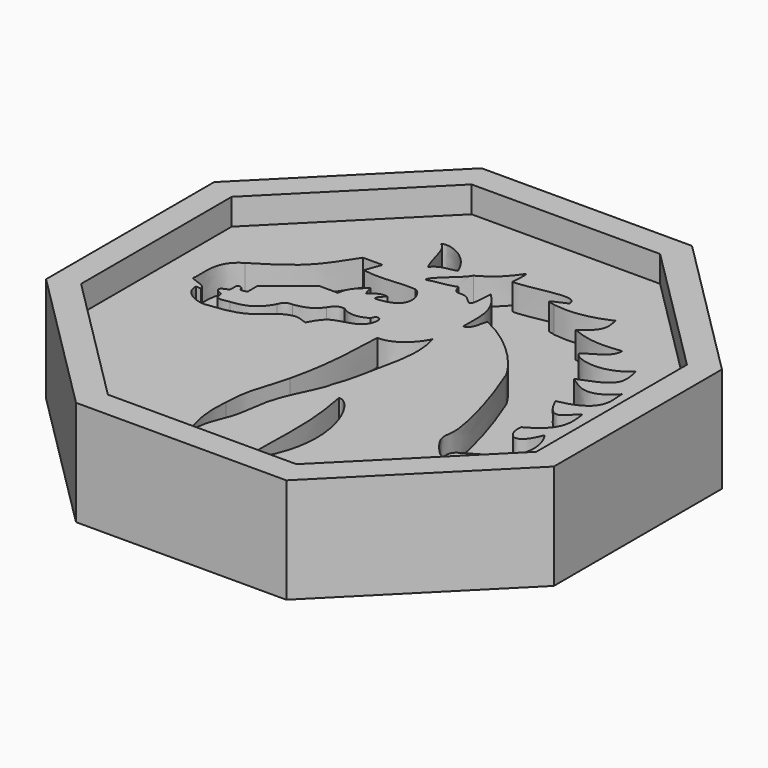
from build123d import *

# Parameters (mm, degrees)
F1_DEPTH = 25.4
F3_DEPTH = 6.35
F5_DEPTH = 6.35


with BuildPart() as f1:
    # F0 (on Top) → F1 (new body)
    with BuildSketch(Plane.XY):
        Polygon((-61.3372846899, 25.3607087968), (-61.3047391097, -25.4392807779), (-25.3607087968, -61.3372846899), (25.4392807779, -61.3047391097), (61.3372846899, -25.3607087968), (61.3047391097, 25.4392807779), (25.3607087968, 61.3372846899), (-25.4392807779, 61.3047391097), align=None)
    extrude(amount=F1_DEPTH)

    # F2 (on face) → F3 (cut)
    with BuildSketch(Plane.XY.offset(25.4)):
        Polygon((-54.9856008905, 22.734521413), (-54.9564255154, -22.8049569991), (-22.734521413, -54.9856008905), (22.8049569991, -54.9564255154), (54.9856008905, -22.734521413), (54.9564255154, 22.8049569991), (22.734521413, 54.9856008905), (-22.8049569991, 54.9564255154), align=None)
    extrude(amount=-F3_DEPTH, mode=Mode.SUBTRACT)

    # F4 (on face) → F5 (cut)
    with BuildSketch(Plane.XY.offset(19.05)):
        with BuildLine():
            add(Edge.make_bspline(
                [(-5.153701175, 4.4508399442), (-0.833334052, 4.1849701665), (2.5564921089, 8.5718045011), (3.3540986478, 10.5658201501)],
                knots=[0, 0, 0, 0, 10.4773871143, 10.4773871143, 10.4773871143, 10.4773871143], degree=3))
            add(Edge.make_bspline(
                [(-5.153701175, 4.4508399442), (-5.4195700213, -3.591689514), (-5.6189713068, -9.9060712382), (-7.679454051, -18.7462065369)],
                knots=[0, 0, 0, 0, 23.3341465033, 23.3341465033, 23.3341465033, 23.3341465033], degree=3))
            add(Edge.make_bspline(
                [(-7.679454051, -18.7462065369), (-9.0719601139, -24.574264884), (-10.8464211226, -26.8810596317), (-11.023866944, -33.9789055288)],
                knots=[0, 0, 0, 0, 15.5955191057, 15.5955191057, 15.5955191057, 15.5955191057], degree=3))
            add(Edge.make_bspline(
                [(-11.023866944, -33.9789055288), (-11.5562053397, -39.74590078), (-10.4887805988, -43.8993513545), (-9.1579346096, -47.1821032425)],
                knots=[0, 0, 0, 0, 13.3343966247, 13.3343966247, 13.3343966247, 13.3343966247], degree=3))
            add(Edge.make_bspline(
                [(-9.1579346096, -47.1821032425), (-8.9959710334, -45.6156823817), (-8.6717623007, -42.2462205811), (-5.5329473264, -35.9645421954), (-5.7178687316, -27.1594780558), (0, -17.6881060287), (0, -15.9681290388)],
                knots=[0, 0, 0, 0, 0.1950520786, 0.422268383, 0.6975815763, 1, 1, 1, 1], degree=3))
            add(Edge.make_bspline(
                [(0, -15.9681290388), (1.8409744371, -11.531976983), (2.5640691165, -5.3227096796), (3.7928808015, 0)],
                knots=[0, 0, 0, 0, 16.4124065808, 16.4124065808, 16.4124065808, 16.4124065808], degree=3))
            add(Edge.make_bspline(
                [(3.3540986478, 10.5658201501), (4.7499099746, 5.580781959), (4.0587496478, 3.0550297815), (3.7928808015, 0)],
                knots=[0, 0, 0, 0, 10.574927197, 10.574927197, 10.574927197, 10.574927197], degree=3))
        make_face()
        with BuildLine():
            add(Edge.make_bspline(
                [(-43.7936633825, 12.6927187666), (-33.5904657841, 18.7789648771), (-32.7022336423, 20.7330770791), (-27.7281291783, 28.312664479)],
                knots=[0, 0, 0, 0, 22.4072330582, 22.4072330582, 22.4072330582, 22.4072330582], degree=3))
            add(Edge.make_bspline(
                [(-43.7936633825, 12.6927187666), (-49.2439717054, 9.5687611029), (-46.8511544168, 3.2543782145), (-47.6487614214, 1.7921003746)],
                knots=[0, 0, 0, 0, 11.5622343091, 11.5622343091, 11.5622343091, 11.5622343091], degree=3))
            add(Edge.make_bspline(
                [(-47.6487614214, 1.7921003746), (-46.3637287418, 0.9944941849), (-43.7936633825, 0.7950926083), (-43.7936633825, -0.6007181946)],
                knots=[0, 0, 0, 0, 4.5373297869, 4.5373297869, 4.5373297869, 4.5373297869], degree=3))
            add(Edge.make_bspline(
                [(-43.7936633825, -0.6007181946), (-44.1924668849, -0.6007181946), (-44.5912703872, -0.6007181946), (-44.9900738895, -0.6007181946)],
                knots=[0, 0, 0, 0, 1.196410507, 1.196410507, 1.196410507, 1.196410507], degree=3))
            add(Edge.make_bspline(
                [(-44.9900738895, -0.6007181946), (-45.1230071485, -4.1899462231), (-40.1379652321, -5.6522237137), (-38.5427549481, -5.1204864867)],
                knots=[0, 0, 0, 0, 7.8737682812, 7.8737682812, 7.8737682812, 7.8737682812], degree=3))
            add(Edge.make_bspline(
                [(-38.5427549481, -5.1204864867), (-27.9080048203, -4.2564133182), (-29.1930399835, -0.9552098345), (-24.451714009, 1.1274284916)],
                knots=[0, 0, 0, 0, 15.4140804566, 15.4140804566, 15.4140804566, 15.4140804566], degree=3))
            add(Edge.make_bspline(
                [(-24.451714009, 1.1274284916), (-21.6600932181, 2.25737039), (-21.2264427294, 1.0571385501), (-19.6755416691, 0.8798926719)],
                knots=[0, 0, 0, 0, 4.7825825871, 4.7825825871, 4.7825825871, 4.7825825871], degree=3))
            add(Edge.make_bspline(
                [(-19.6755416691, 0.8798926719), (-17.4190271646, 5.053767818), (-16.5865225717, 4.7882171348), (-13.464611955, 5.7733519934)],
                knots=[0, 0, 0, 0, 7.9070596333, 7.9070596333, 7.9070596333, 7.9070596333], degree=3))
            add(Edge.make_bspline(
                [(-13.464611955, 5.7733519934), (-9.7631495446, 6.7144022323), (-9.5122028142, 9.0983957052), (-9.4494661316, 9.9139725789)],
                knots=[0, 0, 0, 0, 5.7676801936, 5.7676801936, 5.7676801936, 5.7676801936], degree=3))
            add(Edge.make_bspline(
                [(-9.4494661316, 9.9139725789), (-9.5130050048, 10.6128992403), (-10.0662827589, 11.2702429195), (-11.0193404401, 10.7820779901), (-11.1433556303, 9.9139725789)],
                knots=[0, 0, 0, 0, 0.4822181439, 1, 1, 1, 1], degree=3))
            add(Edge.make_bspline(
                [(-11.1433556303, 9.9139725789), (-12.0216691867, 9.4748158008), (-14.7193456069, 7.9063987359), (-17.4170229584, 9.9139725789)],
                knots=[0, 0, 0, 0, 6.2736673281, 6.2736673281, 6.2736673281, 6.2736673281], degree=3))
            add(Edge.make_bspline(
                [(-17.4170229584, 9.9139725789), (-18.2325989008, 9.9139725789), (-19.1109124571, 10.2903926745), (-20.4283818603, 8.1573463976)],
                knots=[0, 0, 0, 0, 3.4862613179, 3.4862613179, 3.4862613179, 3.4862613179], degree=3))
            add(Edge.make_bspline(
                [(-20.4283818603, 8.1573463976), (-21.745853126, 6.2752454542), (-23.3142692596, 5.5224061944), (-26.137419045, 5.0832494162)],
                knots=[0, 0, 0, 0, 6.4840710844, 6.4840710844, 6.4840710844, 6.4840710844], degree=3))
            add(Edge.make_bspline(
                [(-26.137419045, 5.0832494162), (-27.1412041038, 5.1459865645), (-28.144992888, 4.6440928709), (-28.5214129835, 3.3893594518)],
                knots=[0, 0, 0, 0, 2.9244983007, 2.9244983007, 2.9244983007, 2.9244983007], degree=3))
            add(Edge.make_bspline(
                [(-28.5214129835, 3.3893594518), (-30.5917225778, -0.5003142287), (-33.2266651094, -1.12768088), (-36.0498130322, -1.441364293)],
                knots=[0, 0, 0, 0, 8.9449817882, 8.9449817882, 8.9449817882, 8.9449817882], degree=3))
            add(Edge.make_bspline(
                [(-36.0498130322, -1.441364293), (-37.4036222083, -1.7066936684), (-39.5547804741, -2.1193183366), (-39.0422801094, 0.3359437743), (-40.8038466022, 0.3445137653), (-41.1962555545, 1.9460313525), (-38.8704378187, 2.1547470128), (-39.2634177998, 3.7380327234), (-39.1247228012, 4.7924157188), (-37.7836521987, 4.5584381006), (-37.7563586264, 3.2850185978), (-36.639120561, 3.6665562247), (-36.0498130322, 3.8912522141)],
                knots=[0, 0, 0, 0, 0.1488425547, 0.2535303118, 0.353105288, 0.4397851276, 0.5520245867, 0.6506971423, 0.7299289356, 0.813954275, 0.8940290279, 1, 1, 1, 1], degree=3))
            add(Edge.make_bspline(
                [(-36.0498130322, 3.8912522141), (-36.0498130322, 4.7486534653), (-36.0498130322, 5.9197376637), (-36.0498130322, 6.7771389149)],
                knots=[0, 0, 0, 0, 2.8858867008, 2.8858867008, 2.8858867008, 2.8858867008], degree=3))
            add(Edge.make_bspline(
                [(-36.0498130322, 6.7771389149), (-32.9757171373, 9.3284300528), (-30.0270927449, 11.5660382435), (-26.95299685, 14.1173293814)],
                knots=[0, 0, 0, 0, 11.6889033162, 11.6889033162, 11.6889033162, 11.6889033162], degree=3))
            add(Edge.make_bspline(
                [(-26.95299685, 14.1173293814), (-25.3845794747, 14.1173293814), (-23.9938100179, 14.1173293814), (-22.4253926426, 14.1173293814)],
                knots=[0, 0, 0, 0, 4.5276042074, 4.5276042074, 4.5276042074, 4.5276042074], degree=3))
            add(Edge.make_bspline(
                [(-22.4253926426, 14.1173293814), (-22.2210865468, 17.0617159456), (-19.9708938599, 18.3644555509), (-18.9050156623, 19.489550963)],
                knots=[0, 0, 0, 0, 6.4229135761, 6.4229135761, 6.4229135761, 6.4229135761], degree=3))
            add(Edge.make_bspline(
                [(-18.9050156623, 19.489550963), (-18.5299832374, 18.8184417784), (-18.5102447867, 17.910471186), (-18.1352123618, 17.2393620014)],
                knots=[0, 0, 0, 0, 2.3782235985, 2.3782235985, 2.3782235985, 2.3782235985], degree=3))
            add(Edge.make_bspline(
                [(-18.1352123618, 17.2393620014), (-17.1285495162, 18.5421034694), (-14.9967903271, 19.1342588514), (-14.226987958, 18.7789648771)],
                knots=[0, 0, 0, 0, 4.2005469889, 4.2005469889, 4.2005469889, 4.2005469889], degree=3))
            add(Edge.make_bspline(
                [(-14.226987958, 18.7789648771), (-14.6809735646, 18.0683787912), (-15.5889447778, 18.0091634393), (-15.5889447778, 16.6472066194)],
                knots=[0, 0, 0, 0, 2.5296876583, 2.5296876583, 2.5296876583, 2.5296876583], degree=3))
            add(Edge.make_bspline(
                [(-11.8583673611, 24.4044419378), (-10.081901215, 23.8122865558), (-6.5881847404, 17.1209294349), (-15.5889447778, 16.6472066194)],
                knots=[0, 0, 0, 0, 8.6076656329, 8.6076656329, 8.6076656329, 8.6076656329], degree=3))
            add(Edge.make_bspline(
                [(-24.4120582938, 24.4044419378), (-19.3195231259, 23.575425148), (-16.0034541041, 24.7597359121), (-11.8583673611, 24.4044419378)],
                knots=[0, 0, 0, 0, 12.5536909327, 12.5536909327, 12.5536909327, 12.5536909327], degree=3))
            add(Edge.make_bspline(
                [(-22.990886122, 28.312664479), (-23.4646101793, 27.069138363), (-23.9383342365, 25.6479680538), (-24.4120582938, 24.4044419378)],
                knots=[0, 0, 0, 0, 4.1585975729, 4.1585975729, 4.1585975729, 4.1585975729], degree=3))
            add(Edge.make_bspline(
                [(-27.7281291783, 28.312664479), (-26.1490481595, 28.312664479), (-24.5699671408, 28.312664479), (-22.990886122, 28.312664479)],
                knots=[0, 0, 0, 0, 4.7372430563, 4.7372430563, 4.7372430563, 4.7372430563], degree=3))
        make_face()
        with BuildLine():
            add(Edge.make_bspline(
                [(-15.768840909, 33.0073982477), (-17.3892267048, 35.9319970012), (-17.5473131239, 40.9117229283), (-19.7210032493, 41.8207198381)],
                knots=[0, 0, 0, 0, 9.6588935505, 9.6588935505, 9.6588935505, 9.6588935505], degree=3))
            add(Edge.make_bspline(
                [(-15.768840909, 33.0073982477), (-14.1879757866, 34.9834784865), (-12.1460252752, 34.6146101753), (-10.3543782607, 35.2996513247)],
                knots=[0, 0, 0, 0, 5.8796964156, 5.8796964156, 5.8796964156, 5.8796964156], degree=3))
            add(Edge.make_bspline(
                [(-19.7210032493, 41.8207198381), (-19.3662596851, 42.2371880653), (-16.8995265641, 42.4462175322), (-12.0895465268, 39.5981340454), (-10.3543782607, 35.2996513247)],
                knots=[0, 0, 0, 0, 0.3200449041, 1, 1, 1, 1], degree=3))
        make_face()
        with BuildLine():
            add(Edge.make_bspline(
                [(-12.9232844338, 29.0552340448), (-12.0142865926, 30.9522729367), (-8.4178196266, 33.0864414573), (-6.8764751777, 35.5763025582)],
                knots=[0, 0, 0, 0, 8.8931567363, 8.8931567363, 8.8931567363, 8.8931567363], degree=3))
            add(Edge.make_bspline(
                [(-12.9232844338, 29.0552340448), (-12.9232844338, 28.9234953622), (-12.9232844338, 28.7917566796), (-12.9232844338, 28.660017997)],
                knots=[0, 0, 0, 0, 0.3952160478, 0.3952160478, 0.3952160478, 0.3952160478], degree=3))
            add(Edge.make_bspline(
                [(-12.9232844338, 28.660017997), (-10.4447612539, 29.4240117073), (-8.1823244691, 29.3352883309), (-6.1650867574, 30.2804056555)],
                knots=[0, 0, 0, 0, 6.9497404266, 6.9497404266, 6.9497404266, 6.9497404266], degree=3))
            add(Edge.make_bspline(
                [(-6.1650867574, 30.2804056555), (-5.9334094435, 29.4659731174), (-5.4670946491, 27.8370222868), (-2.5904509764, 28.8559552397), (0.264793503, 24.5950136707), (0.2685460786, 28.8916733116), (0.468172424, 31.6864475608)],
                knots=[0, 0, 0, 0, 0.2064192131, 0.4285927417, 0.6702836236, 1, 1, 1, 1], degree=3))
            add(Edge.make_bspline(
                [(0.468172424, 31.6864475608), (5.5923829786, 26.7663598061), (4.4173980132, 22.5834138691), (4.55839606, 18.1184709072)],
                knots=[0, 0, 0, 0, 14.1710945189, 14.1710945189, 14.1710945189, 14.1710945189], degree=3))
            add(Edge.make_bspline(
                [(4.55839606, 18.1184709072), (6.8143671378, 18.8704598695), (6.219041689, 21.0324327151), (7.0493645035, 22.489413619)],
                knots=[0, 0, 0, 0, 5.0309108496, 5.0309108496, 5.0309108496, 5.0309108496], degree=3))
            add(Edge.make_bspline(
                [(7.0493645035, 22.489413619), (14.9920871481, 18.9425181597), (21.1890060455, 11.6893071681), (23.2311710715, 7.8866528347)],
                knots=[0, 0, 0, 0, 21.796593457, 21.796593457, 21.796593457, 21.796593457], degree=3))
            add(Edge.make_bspline(
                [(23.2311710715, 7.8866528347), (24.3144150819, 5.142826258), (26.7466632507, -1.016760046), (31.0793052513, -16.4688597233), (28.7968482547, -20.1379000544), (35.154530862, -27.1249514355), (34.8396243261, -24.4686414852), (35.2501716709, -22.4396670807), (46.1667067572, -18.2589361031), (46.4346853173, -10.7153912499), (45.065808231, -7.9198662645), (44.3560816348, -6.8906880915)],
                knots=[0, 0, 0, 0, 0.1439636646, 0.3208577525, 0.415015494, 0.5337685413, 0.5809072881, 0.6428347208, 0.7904691121, 0.9075491711, 1, 1, 1, 1], degree=3))
            add(Edge.make_bspline(
                [(38.8290174305, -7.1419184096), (38.2846854627, -10.8684999868), (41.6886657476, -14.2322224565), (44.3560816348, -6.8906880915)],
                knots=[0, 0, 0, 0, 5.5327710408, 5.5327710408, 5.5327710408, 5.5327710408], degree=3))
            add(Edge.make_bspline(
                [(38.8290174305, -7.1419184096), (46.0728220642, -3.3315932378), (45.0260303915, 0.5624747719), (44.6910560131, 3.9959545247)],
                knots=[0, 0, 0, 0, 12.5863302771, 12.5863302771, 12.5863302771, 12.5863302771], degree=3))
            add(Edge.make_bspline(
                [(44.6910560131, 3.9959545247), (43.0580601096, 3.9959545247), (40.9822575748, -3.171547316), (37.2556746006, 5.2446648479)],
                knots=[0, 0, 0, 0, 7.5395075582, 7.5395075582, 7.5395075582, 7.5395075582], degree=3))
            add(Edge.make_bspline(
                [(37.2556746006, 5.2446648479), (48.1260122449, 7.3031691768), (44.8868456619, 13.2512337448), (45.3151115595, 15.2979912768)],
                knots=[0, 0, 0, 0, 12.8850260528, 12.8850260528, 12.8850260528, 12.8850260528], degree=3))
            add(Edge.make_bspline(
                [(34.2816302428, 14.5025634131), (36.4091768861, 13.2117252797), (39.7951751947, 9.3775773421), (45.3151115595, 15.2979912768)],
                knots=[0, 0, 0, 0, 11.0621162284, 11.0621162284, 11.0621162284, 11.0621162284], degree=3))
            add(Edge.make_bspline(
                [(34.2816302428, 14.5025634131), (37.4293167665, 15.6832908865), (43.070982412, 17.7995339028), (42.0079146419, 22.1456028948), (41.5379703045, 24.0668449551)],
                knots=[0, 0, 0, 0, 0.5579356739, 1, 1, 1, 1], degree=3))
            add(Edge.make_bspline(
                [(28.5914987326, 23.1207553297), (29.3384101242, 21.2285798043), (36.3095887005, 19.2368142307), (41.5379703045, 24.0668449551)],
                knots=[0, 0, 0, 0, 12.9809942509, 12.9809942509, 12.9809942509, 12.9809942509], degree=3))
            add(Edge.make_bspline(
                [(28.5914987326, 23.1207553297), (30.5002729098, 25.0959228724), (34.3178212643, 25.6602559239), (34.3178212643, 29.0462579578)],
                knots=[0, 0, 0, 0, 8.2402882918, 8.2402882918, 8.2402882918, 8.2402882918], degree=3))
            add(Edge.make_bspline(
                [(22.0421720296, 30.3383134305), (27.1474681795, 28.199756518), (30.4338801652, 28.647903353), (34.3178212643, 29.0462579578)],
                knots=[0, 0, 0, 0, 12.3434586513, 12.3434586513, 12.3434586513, 12.3434586513], degree=3))
            add(Edge.make_bspline(
                [(22.0421720296, 30.3383134305), (26.9771087915, 33.5342735052), (25.9901210666, 35.4142487049), (25.6141256541, 37.9522144794)],
                knots=[0, 0, 0, 0, 8.4101332854, 8.4101332854, 8.4101332854, 8.4101332854], degree=3))
            add(Edge.make_bspline(
                [(12.4072954059, 35.7902422547), (18.0002246052, 35.0852534175), (21.807173267, 36.2602360547), (25.6141256541, 37.9522144794)],
                knots=[0, 0, 0, 0, 13.3826189181, 13.3826189181, 13.3826189181, 13.3826189181], degree=3))
            add(Edge.make_bspline(
                [(14.3812708557, 37.9992127419), (13.4644072953, 37.5805370404), (11.9867321494, 37.0078461454), (10.3610867603, 36.0403140522), (11.8929853111, 36.0695067901), (12.4072954059, 35.7902422547)],
                knots=[0, 0, 0, 0, 0.4317345562, 0.6867739539, 1, 1, 1, 1], degree=3))
            add(Edge.make_bspline(
                [(0.468172424, 38.2308661938), (5.2468694824, 38.0909827848), (14.663268812, 41.8531633914), (14.3812708557, 37.9992127419)],
                knots=[0, 0, 0, 0, 13.915026816, 13.915026816, 13.915026816, 13.915026816], degree=3))
            add(Edge.make_bspline(
                [(0, 41.7416766286), (0.1797526793, 42.0766967821), (0.771681502, 43.179924204), (0.5927601967, 40.2624104176), (0.468172424, 38.2308661938)],
                knots=[0, 0, 0, 0, 0.3036727938, 1, 1, 1, 1], degree=3))
            add(Edge.make_bspline(
                [(-6.8764751777, 35.5763025582), (-3.3590511885, 37.4733395874), (-1.8572298577, 39.2122901976), (0, 41.7416766286)],
                knots=[0, 0, 0, 0, 9.2356780096, 9.2356780096, 9.2356780096, 9.2356780096], degree=3))
        make_face()
        with BuildLine():
            add(Edge.make_bspline(
                [(4.5185703784, -19.2535147071), (7.8085283749, -18.5015238822), (17.3964034766, -35.2333076298), (6.0225501657, -50.3671132028)],
                knots=[0, 0, 0, 0, 31.1499272319, 31.1499272319, 31.1499272319, 31.1499272319], degree=3))
            add(Edge.make_bspline(
                [(4.5185703784, -19.2535147071), (7.1505359374, -31.8493526429), (5.4585578231, -39.8079163084), (6.0225501657, -50.3671132028)],
                knots=[0, 0, 0, 0, 31.1499272319, 31.1499272319, 31.1499272319, 31.1499272319], degree=3))
        make_face()
    extrude(amount=-F5_DEPTH, mode=Mode.SUBTRACT)


solid = f1.part
